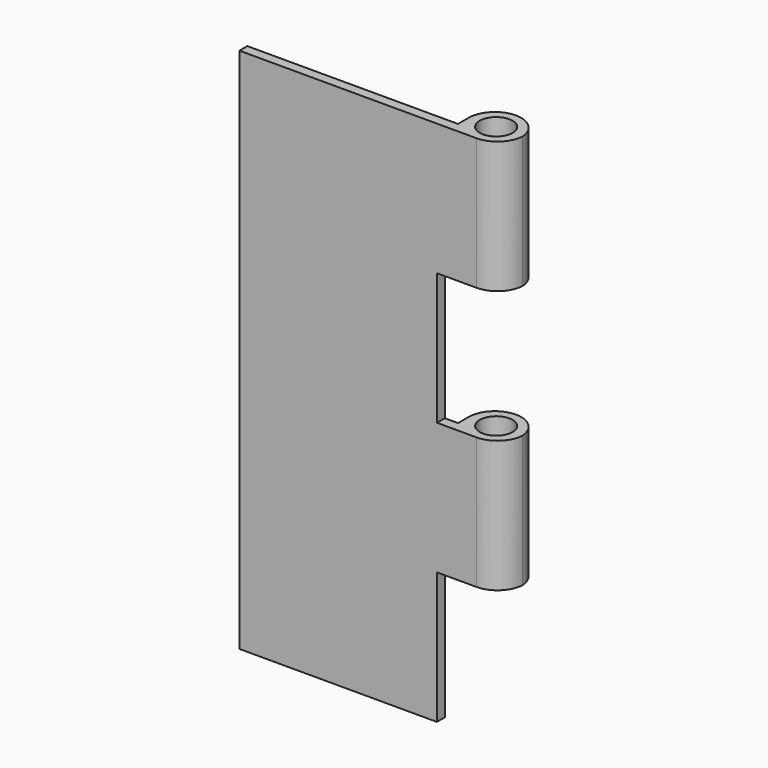
from build123d import *

# Parameters (mm, degrees)
F0_W        = 12.7
F0_H        = 25.4
F1_DEPTH    = 9.525
F2_T1_DEPTH = 50.8
F2_T3_DEPTH = 50.8
F3_R        = 3.175
F4_DEPTH    = 101.601
F5_W        = 40.64
F5_H        = 7.62
F6_DEPTH    = 101.601
F7_R        = 5.07999


# Not quite as in the source:
# - a fillet or chamfer that OpenCascade refuses, or shapes differently, is made with other operations: its cross-section is extruded or revolved along the edge and cut away or added
# - a fillet or chamfer is up to 0.001 mm smaller than in the source, because OpenCascade refuses the exact size


with BuildPart() as f1:
    # F0 (on Front) → F1 (new body)
    with BuildSketch(Plane.XZ):
        with Locations((19.05, 38.1)):
            Rectangle(F0_W, F0_H)
        Polygon((12.7, 25.4), (12.7, 50.8), (-25.4, 50.8), (-25.4, -50.8), (12.7, -50.8), (12.7, -25.4), (12.7, 0), align=None)
        with Locations((19.05, -12.7)):
            Rectangle(F0_W, F0_H)
    extrude(amount=F1_DEPTH)

    # F2: fillet of radius 5.08 on 4 edges, made by hand

    # F2_s2 → F2_t1 (cut)
    with BuildSketch(Plane.XY.offset(12.7)):
        with BuildLine():
            ThreePointArc((25.4, -5.08), (23.9121024484, -1.4878975516), (20.32, 0))
            Line((20.32, 0), (25.4, 0))
            Line((25.4, 0), (25.4, -5.08))
        make_face()
        with BuildLine():
            ThreePointArc((25.4, -4.445), (23.9121024484, -8.0371024484), (20.32, -9.525))
            Line((20.32, -9.525), (25.4, -9.525))
            Line((25.4, -9.525), (25.4, -4.445))
        make_face()
    extrude(amount=F2_T1_DEPTH, mode=Mode.SUBTRACT)

    # F2_s4 → F2_t3 (cut)
    with BuildSketch(Plane.XY.offset(-38.1)):
        with BuildLine():
            ThreePointArc((25.4, -5.08), (23.9121024484, -1.4878975516), (20.32, 0))
            Line((20.32, 0), (25.4, 0))
            Line((25.4, 0), (25.4, -5.08))
        make_face()
        with BuildLine():
            ThreePointArc((25.4, -4.445), (23.9121024484, -8.0371024484), (20.32, -9.525))
            Line((20.32, -9.525), (25.4, -9.525))
            Line((25.4, -9.525), (25.4, -4.445))
        make_face()
    extrude(amount=F2_T3_DEPTH, mode=Mode.SUBTRACT)

    # F3 (on face) → F4 (cut, through all)
    with BuildSketch(Plane.XY.offset(50.8)):
        with Locations((20.32, -4.7625)):
            Circle(F3_R)
    extrude(amount=-F4_DEPTH, mode=Mode.SUBTRACT)

    # F5 (on face) → F6 (cut, through all)
    with BuildSketch(Plane.XY.offset(50.8)):
        with Locations((-5.08, -3.81)):
            Rectangle(F5_W, F5_H)
    extrude(amount=-F6_DEPTH, mode=Mode.SUBTRACT)

    # F7 (radius 5.08 in the source; OpenCascade refuses exactly that, so slightly less here)
    f7_edges = [f1.edges().sort_by_distance(p)[0] for p in [
        (15.24, 0, 38.1),
        (15.24, 0, -12.7),
    ]]
    fillet(f7_edges, radius=F7_R)


solid = f1.part
